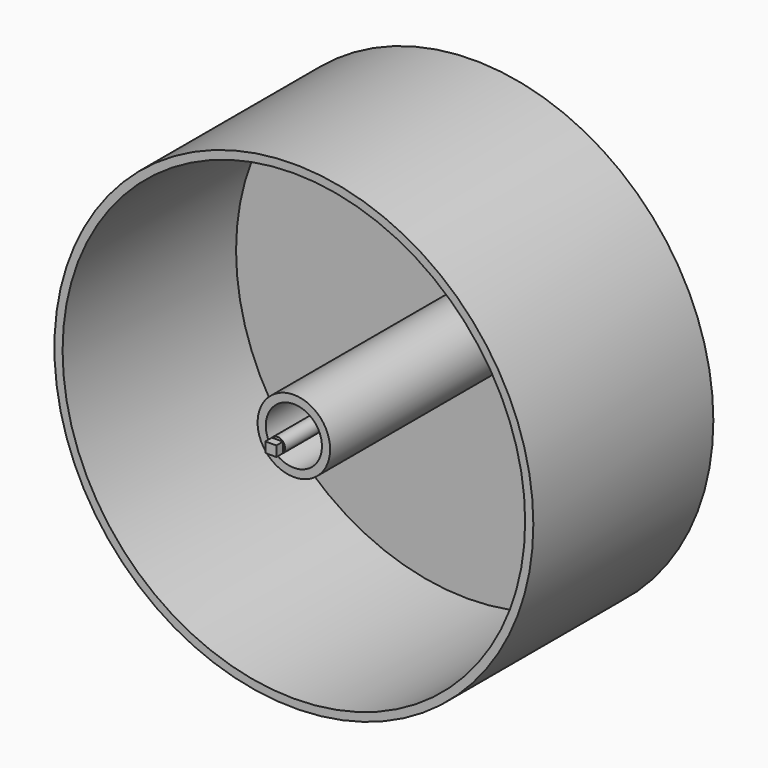
from build123d import *

# Parameters (mm, degrees)
F0_R     = 74.3348604036
F1_DEPTH = 69.85
F2_T     = -2.54
F3_R     = 11.2538360461
F4_DEPTH = 67.31
F5_T     = -2.54
F6_R     = 2.3281724299
F7_DEPTH = 73.66
F9_DEPTH = 2.54


# Not quite as in the source:
# - a shell that OpenCascade refuses in one call is made with other operations: the cavity is built on its own and cut out


with BuildPart() as f1:
    # F0 (on Front) → F1 (new body)
    with BuildSketch(Plane.XZ):
        Circle(F0_R)
    extrude(amount=F1_DEPTH)

    # F2
    f2_openings = [f1.faces().sort_by_distance(p)[0] for p in [
        (0, -69.85, 0),
    ]]
    offset(amount=F2_T, openings=f2_openings)

    # F3 (on face) → F4 (join)
    with BuildSketch(Plane.XZ.offset(2.54)):
        Circle(F3_R)
    extrude(amount=F4_DEPTH)

    # F5: a shell. OpenCascade refuses it in one call, so the cavity is built on its own and cut out:
    # the body offset inwards by the wall thickness, plus a prism from it out through each open face.
    f5_core = offset(f1.part, amount=F5_T, kind=Kind.INTERSECTION, mode=Mode.PRIVATE)
    f5_exits = [f5_core.faces().sort_by_distance(p)[0] for p in [
        (0, -67.31, 0),
    ]]
    add(f5_core, mode=Mode.SUBTRACT)
    extrude(f5_exits, amount=-F5_T, mode=Mode.SUBTRACT)

    # F6 (on face) → F7 (join)
    with BuildSketch(Plane.XZ.offset(2.54)):
        Circle(F6_R)
    extrude(amount=F7_DEPTH)

    # F8 (on face) → F9 (join)
    with BuildSketch(Plane.XZ.offset(76.2)):
        with BuildLine():
            Line((1.6746039799, 1.552517079), (-1.7349575161, 1.552517079))
            Line((-1.7349575161, 1.552517079), (-1.7349575161, -1.552517079))
            ThreePointArc((-1.7349575161, -1.552517079), (-1.7050897064, -1.5852621097), (-1.6746039799, -1.6174326489))
            Line((-1.6746039799, -1.6174326489), (1.6746039799, -1.6174326489))
            Line((1.6746039799, -1.6174326489), (1.6746039799, 1.552517079))
        make_face()
    extrude(amount=F9_DEPTH)


solid = f1.part
